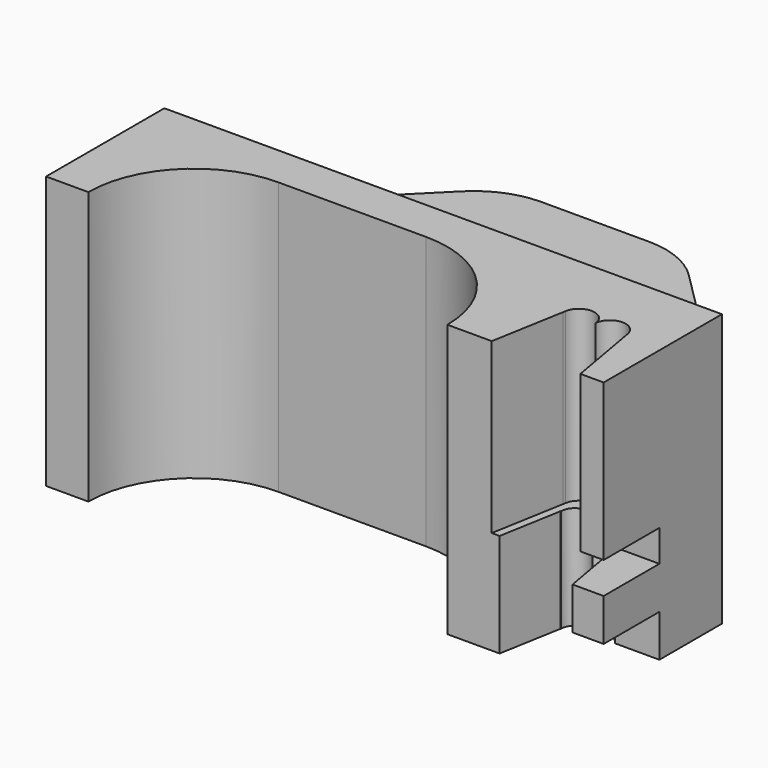
from build123d import *

# Parameters (mm, degrees)
F1_DEPTH  = 16.383
F2_W      = 33.528
F2_H      = 5.969
F3_DEPTH  = 11.43
F4_SIZE   = 11.43
F5_R      = 2.159
F6_DEPTH  = 25.4
F8_DEPTH  = 6.35
F10_DEPTH = 10.16
F11_R     = 6.34999
F12_W     = 4.191
F12_H     = 2.54
F12_H_2   = 1.905
F13_DEPTH = 2.667
F14_R     = 5.08


# Not quite as in the source:
# - a fillet or chamfer is up to 0.001 mm smaller than in the source, because OpenCascade refuses the exact size


with BuildPart() as f1:
    # F0 (on Top) → F1 (new body)
    with BuildSketch(Plane.XY):
        Polygon((21.1023603916, 14.8059087365), (-12.4256396084, 14.8059087365), (-12.4256396084, 5.9159087365), (-9.8856396084, 5.9159087365), (-9.8856396084, 12.2659087365), (11.7043603916, 12.2659087365), (11.7043603916, 5.9159087365), (21.1023603916, 5.9159087365), align=None)
    extrude(amount=F1_DEPTH)

    # F2 (on face) → F3 (join)
    with BuildSketch(Plane(origin=(0, 14.8059087365, 0), x_dir=(-1, 0, 0), z_dir=(0, 1, 0))):
        with Locations((-4.3383603916, 8.1915)):
            Rectangle(F2_W, F2_H)
    extrude(amount=F3_DEPTH)

    # F4
    f4_edges = [f1.edges().sort_by_distance(p)[0] for p in [
        (-12.42564, 26.235909, 8.1915),
        (21.10236, 26.235909, 8.1915),
    ]]
    chamfer(f4_edges, length=F4_SIZE)

    # F5 (on face) → F6 (cut)
    with BuildSketch(Plane(origin=(0, 0, 5.207), x_dir=(1, 0, 0), z_dir=(0, 0, -1))):
        with Locations((4.3383603916, -19.8859087365)):
            Circle(F5_R)
    extrude(amount=-F6_DEPTH, mode=Mode.SUBTRACT)

    # F7 (on face) → F8 (cut)
    with BuildSketch(Plane(origin=(0, 0, 0), x_dir=(1, 0, 0), z_dir=(0, 0, -1))):
        with BuildLine():
            Line((18.5677868823, -9.6751087365), (19.2306352681, -5.9159087365))
            Line((19.2306352681, -5.9159087365), (14.846085515, -5.9159087365))
            Line((14.846085515, -5.9159087365), (15.5089339009, -9.6751087365))
            Line((15.5089339009, -9.6751087365), (15.5218644869, -9.6751087365))
            ThreePointArc((15.5218644869, -9.6751087365), (16.101190374, -10.4723310604), (17.0383603916, -10.1675454388))
            ThreePointArc((17.0383603916, -10.1675454388), (17.9755304092, -10.4723310604), (18.5548562962, -9.6751087365))
            Line((18.5548562962, -9.6751087365), (18.5677868823, -9.6751087365))
        make_face()
    extrude(amount=-F8_DEPTH, mode=Mode.SUBTRACT)

    # F9 (on face) → F10 (cut)
    with BuildSketch(Plane.XY.offset(16.383)):
        with BuildLine():
            Line((14.3731213639, 5.9159087365), (19.7035994193, 5.9159087365))
            Line((19.7035994193, 5.9159087365), (18.9287834006, 10.3101087365))
            Line((18.9287834006, 10.3101087365), (18.9070608822, 10.4264149788))
            ThreePointArc((18.9070608822, 10.4264149788), (17.9577526403, 11.2497597634), (17.0383603916, 10.3931381052))
            ThreePointArc((17.0383603916, 10.3931381052), (16.1426669703, 11.2490386173), (15.1767129861, 10.4733032939))
            Line((15.1767129861, 10.4733032939), (15.1479373825, 10.3101087365))
            Line((15.1479373825, 10.3101087365), (14.3731213639, 5.9159087365))
        make_face()
    extrude(amount=-F10_DEPTH, mode=Mode.SUBTRACT)

    # F11 (radius 6.35 in the source; OpenCascade refuses exactly that, so slightly less here)
    f11_edges = [f1.edges().sort_by_distance(p)[0] for p in [
        (11.70436, 12.265909, 8.1915),
        (-9.88564, 12.265909, 8.1915),
    ]]
    fillet(f11_edges, radius=F11_R)

    # F12 (on face) → F13 (cut)
    with BuildSketch(Plane.YZ.offset(21.1023603916)):
        with Locations((8.0114087365, 1.27)):
            Rectangle(F12_W, F12_H)
        with Locations((8.0114087365, 6.0325)):
            Rectangle(F12_W, F12_H_2)
    extrude(amount=-F13_DEPTH, mode=Mode.SUBTRACT)

    # F14
    f14_edges = [f1.edges().sort_by_distance(p)[0] for p in [
        (9.67236, 26.235909, 8.1915),
        (-0.99564, 26.235909, 8.1915),
    ]]
    fillet(f14_edges, radius=F14_R)


solid = f1.part
